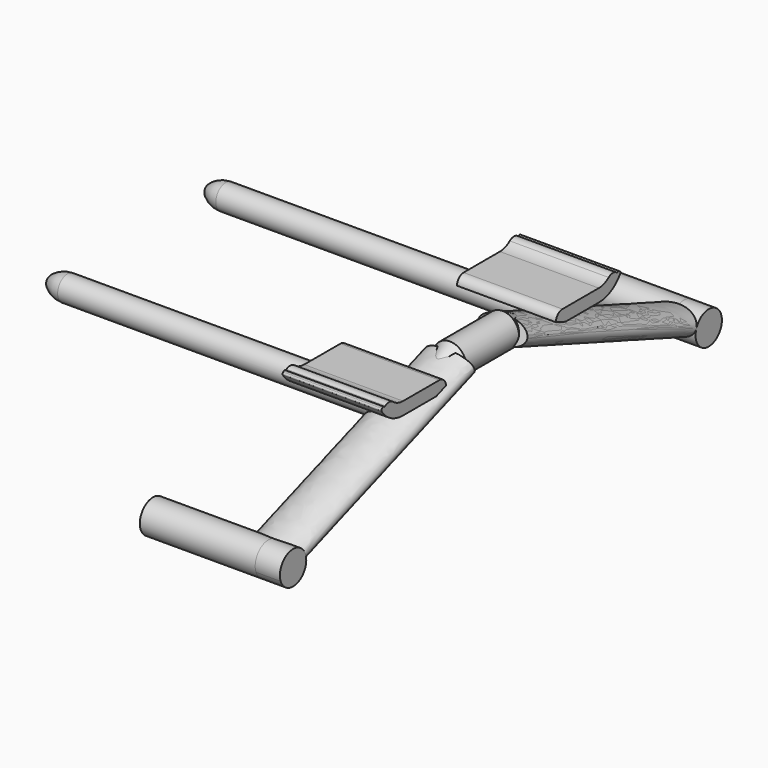
from build123d import *
from build123d import SkipClean  # not in build123d's __all__

# Parameters (mm, degrees)
F1_DEPTH       = 177.8
F2_R           = 12.7
F3_DEPTH       = 19.05
F3_DEPTH_BACK  = 88.9
F8_ANGLE       = -20
F11_R          = 12.7
F12_DEPTH      = 38.1
F12_DEPTH_BACK = 38.1
F13_SIZE2      = 7.3323484187
F13_SIZE       = 12.7
F15_W          = 254
F15_H          = 9.525
F20_DEPTH      = 76.2


# Not quite as in the source:
# - ends of sketch curves that miss each other by under 0.0002 mm in the source are joined
# - a feature names something its author has since deleted; it is built from what else it names
# - the program builds the solid bodies; features that only make, move or delete a surface that nothing else refers to are left out


with BuildPart() as f1:
    # F0 (on Front) → F1 (new body)
    with BuildSketch(Plane.XZ):
        with BuildLine():
            add(Edge.make_bspline(
                [(19.05, 0), (19.05, 16.4977839421), (-9.525, 8.248891971), (-38.1, 0), (-9.525, -8.248891971), (19.05, -16.4977839421), (19.05, 0)],
                knots=[0, 0, 0, 2.0943951024, 2.0943951024, 4.1887902048, 4.1887902048, 6.2831853072, 6.2831853072, 6.2831853072], degree=2, weights=[1, 0.5, 1, 0.5, 1, 0.5, 1]))
        make_face()
    extrude(amount=F1_DEPTH)

    # F2 (on Right) → F3 (join, two sides)
    with BuildSketch(Plane.YZ) as f3_sk:
        with Locations((8.2287123548, 0)):
            Circle(F2_R)
    with SkipClean():  # cleaning this boolean's faces spoils the solid; the shape is the same uncleaned
        extrude(amount=F3_DEPTH)
        extrude(f3_sk.sketch, amount=-F3_DEPTH_BACK)


with BuildPart() as f1_1:
    # F8: moved
    add(f1.part.rotate(Axis((0, -177.8, 0), (1, 0, 0)), F8_ANGLE), clean=False)


with BuildPart() as f10_1:
    # F10: instance of F1
    add(f1_1.part.mirror(Plane.XZ.offset(203.2)), clean=False)

    # F15 (on offset) → F16 (revolve)
    with BuildSketch(Plane.XZ.offset(279.4)):
        with Locations((-127, -8.1803774036)):
            Rectangle(F15_W, F15_H)
        with BuildLine():
            Line((-254, -12.9428774036), (-254, -3.4178774036))
            ThreePointArc((-254, -3.4178774036), (-260.7351920908, -4.6482340991), (-266.6003906189, -8.1803774036))
            ThreePointArc((-266.6003906189, -8.1803774036), (-268.1878906189, -10.3302471973), (-268.7502604126, -12.9428774036))
            Line((-268.7502604126, -12.9428774036), (-254, -12.9428774036))
        make_face()
    revolve(axis=Axis((-106.6287340578, -279.4, -12.9428774036), (-1, 0, 0)))


with BuildPart() as f12:
    # F11 (on offset) → F12 (new body, two sides)
    with BuildSketch(Plane.XZ.offset(203.2)) as f12_sk:
        Circle(F11_R)
    extrude(amount=F12_DEPTH)
    extrude(f12_sk.sketch, amount=-F12_DEPTH_BACK)

    # F13
    f13_edges = [f12.edges().sort_by_distance(p)[0] for p in [
        (12.7, -184.15, 0),
        (-12.7, -203.2, 0),
        (-12.7, -165.1, 0),
        (-12.7, -241.3, 0),
    ]]
    chamfer(f13_edges, length=F13_SIZE, length2=F13_SIZE2)


with BuildPart() as f17_1:
    # F17: instance of F10_1
    add(f10_1.part.mirror(Plane.XZ.offset(203.2)), clean=False)


with BuildPart() as f20:
    # F19 (on offset) → F20 (new body)
    with BuildSketch(Plane.YZ.offset(19.05)):
        with BuildLine():
            ThreePointArc((-318.1431485313, 7.7228010099), (-309.2283973251, -0.4549774235), (-297.4993703883, -3.4178774036))
            Line((-297.4993703883, -3.4178774036), (-265.5473573139, -3.4178774036))
            Line((-265.5473573139, -3.4178774036), (-256.1756968498, 0))
            Line((-256.1756968498, 0), (-297.5191570171, 0.0382599307))
            ThreePointArc((-297.5191570171, 0.0382599307), (-307.6078873139, 2.5786834274), (-315.3033530881, 9.579831165))
            ThreePointArc((-315.3033530881, 9.579831165), (-316.1154993342, 10.1320545436), (-317.0823561313, 9.9596593035))
            Line((-317.0823561313, 9.9596593035), (-317.7500856237, 9.5379983551))
            ThreePointArc((-317.7500856237, 9.5379983551), (-318.3272981434, 8.7128323761), (-318.1431485313, 7.7228010099))
        make_face()
        with BuildLine():
            Line((-297.5191570171, 0.0382599307), (-256.1756968498, 0))
            ThreePointArc((-256.1756968498, 0), (-258.0314127549, 4.4918472938), (-262.5198177369, 6.3558736748))
            Line((-262.5198177369, 6.3558736748), (-297.4993703858, 6.3882443389))
            ThreePointArc((-297.4993703858, 6.3882443389), (-302.5291827612, 7.2547632485), (-306.9790828013, 9.7544146613))
            ThreePointArc((-306.9790828013, 9.7544146613), (-310.680520373, 11.1692100225), (-314.5000587353, 10.1140262898))
            Line((-314.5000587353, 10.1140262898), (-315.3033530881, 9.579831165))
            ThreePointArc((-315.3033530881, 9.579831165), (-307.6078873139, 2.5786834274), (-297.5191570171, 0.0382599307))
        make_face()
    extrude(amount=-F20_DEPTH)


with BuildPart() as f21_1:
    # F21: instance of F20
    add(f20.part.mirror(Plane.XZ.offset(203.2)), clean=False)


solid = Compound([f1_1.part, f10_1.part, f12.part, f17_1.part, f20.part, f21_1.part])
